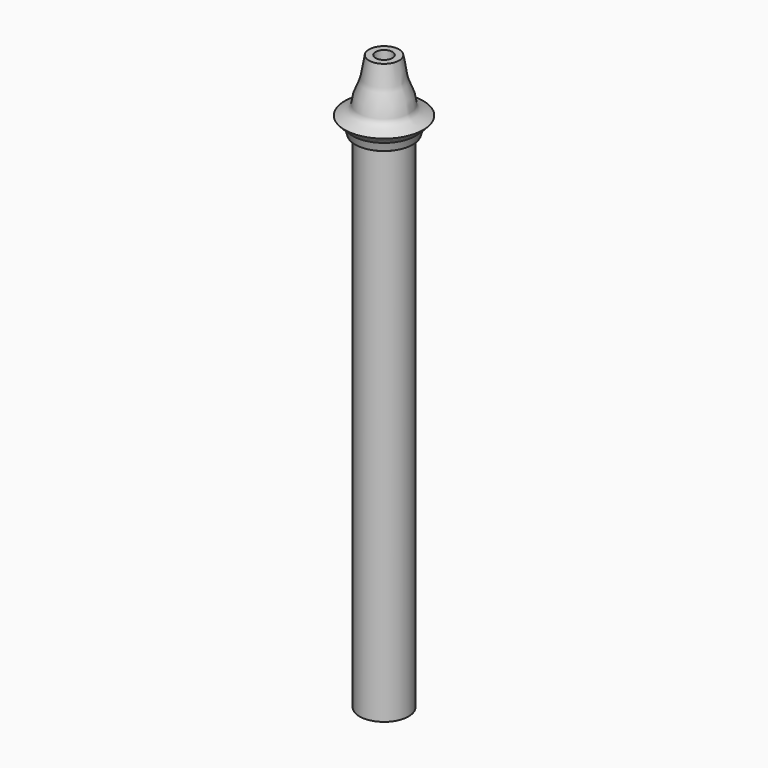
from build123d import *

# Parameters (mm, degrees)
F2_R     = 1.27
F3_DEPTH = 5.08


# Not quite as in the source:
# - a feature names something its author has since deleted; it is built from what else it names


with BuildPart() as f1:
    # F0 (on Front) → F1 (revolve)
    with BuildSketch(Plane.XZ):
        with BuildLine():
            Line((0, 76.2), (0, 0))
            Line((0, 0), (3.683, 0))
            Line((3.683, 0), (3.683, 50.5892820656))
            Line((3.683, 50.5892820656), (3.683, 75.4657239321))
            add(Edge.make_bspline(
                [(3.683, 75.4657239321), (3.9001026563, 75.5844257372), (4.117282526, 75.702956664), (4.3289103642, 75.8188781839)],
                knots=[0, 0, 0, 0, 0.0367930761, 0.0367930761, 0.0367930761, 0.0367930761], degree=3))
            Line((4.3289103642, 75.8188781839), (4.7080438681, 77.083454169))
            Line((4.7080438681, 77.083454169), (5.4083663136, 77.7371979129))
            Line((5.4083663136, 77.7371979129), (5.8970035864, 78.2753947108))
            add(Edge.make_bspline(
                [(5.8970035864, 78.2753947108), (5.4557518487, 78.5243036944), (3.6824791799, 79.0277734306), (3.8959075155, 80.928711884), (2.7015379677, 83.0135115397), (2.599091359, 84.685822435), (2.3724716532, 85.744447935), (2.2606033154, 86.2670275395)],
                knots=[0.4795528936, 0.4795528936, 0.4795528936, 0.4795528936, 0.5884154591, 0.6871467774, 0.8044356188, 0.9034623818, 1, 1, 1, 1], degree=3))
            Line((2.2606033154, 86.2670275395), (0, 86.2670275395))
            Line((0, 86.2670275395), (0, 85.744447935))
            Line((0, 85.744447935), (0, 76.2))
        make_face()
    revolve(axis=Axis((0, 0, 38.1), (0, 0, 1)))

    # F2 (on face) → F3 (cut)
    with BuildSketch(Plane.XY.offset(86.2670275395)):
        Circle(F2_R)
    extrude(amount=-F3_DEPTH, mode=Mode.SUBTRACT)


solid = f1.part
